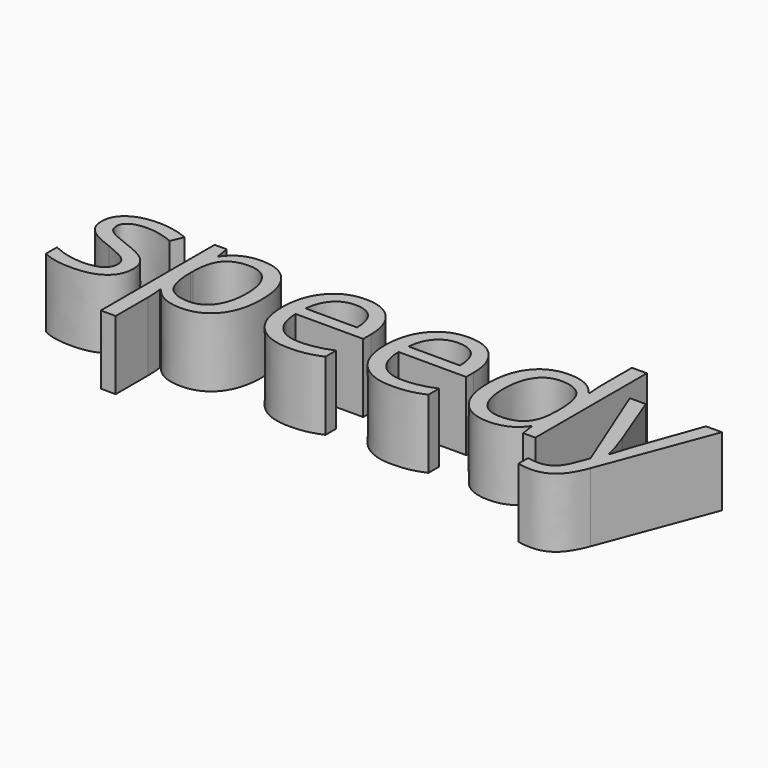
from build123d import *

# Parameters (mm, degrees)
F0_TEXT_SIZE = 77.1555118263
F1_DEPTH     = 28.956


# Not quite as in the source:
# - Text() gives the source's letters only with a copy of the font that has no kerning and outlines rounded to 1/6400 em; it was checked with that copy


with BuildPart() as f1:
    # F0 (on Top) → F1 (new body)
    with BuildSketch(Plane.XY):
        with Locations((-61.4294819534, 0)):
            Text('speedy', F0_TEXT_SIZE, font='Open Sans', text_align=(TextAlign.LEFT, TextAlign.BOTTOM))
    extrude(amount=F1_DEPTH)


solid = f1.part
